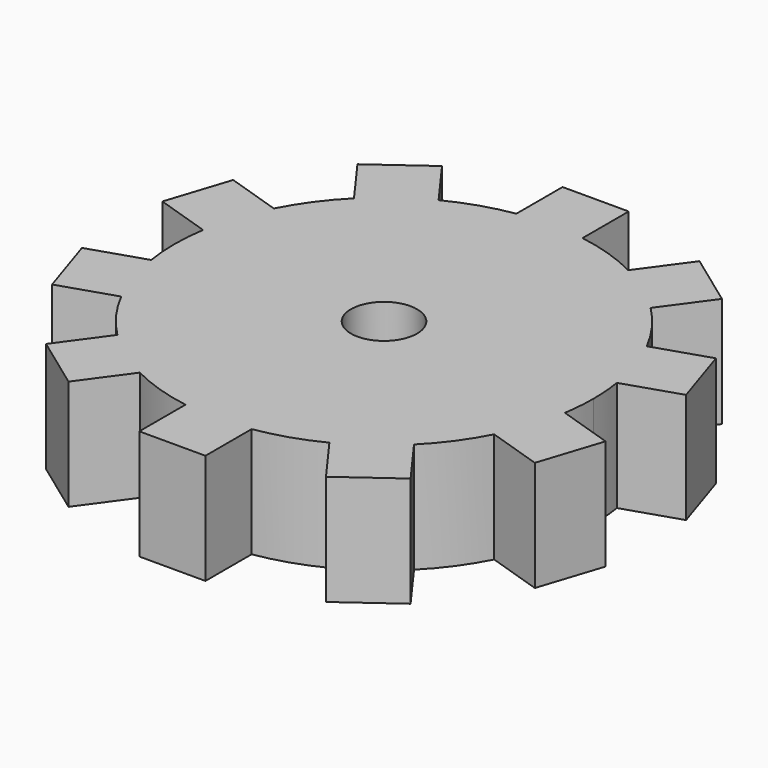
from build123d import *

# Parameters (mm, degrees)
F1_DEPTH = 12.7
F2_R     = 3.81
F3_DEPTH = 25.4


# Not quite as in the source:
# - a feature names something its author has since deleted; it is built from what else it names


with BuildPart() as f1:
    # F0 (on Top) → F1 (new body)
    with BuildSketch(Plane.XY):
        with BuildLine():
            ThreePointArc((23.8384751489, -3.7395190297), (24.0570083899, -1.8754325709), (24.13, 0))
            ThreePointArc((24.13, 0), (24.0570083899, 1.8754325709), (23.8384751489, 3.7395190297))
            Line((23.8384751489, 3.7395190297), (12.3294189943, 0))
            Line((12.3294189943, 0), (23.8384751489, -3.7395190297))
        make_face()
        with BuildLine():
            Line((12.3294189943, 0), (23.8384751489, 3.7395190297))
            ThreePointArc((23.8384751489, 3.7395190297), (22.9489937382, 7.4565800743), (21.4837656518, 10.9865696839))
            Line((21.4837656518, 10.9865696839), (9.9747094971, 7.2470506542))
            Line((9.9747094971, 7.2470506542), (6.1647094971, 2.0030355372))
            Line((6.1647094971, 2.0030355372), (12.3294189943, 0))
        make_face()
        with BuildLine():
            ThreePointArc((21.4837656518, 10.9865696839), (22.9489937382, 7.4565800743), (23.8384751489, 3.7395190297))
            Line((23.8384751489, 3.7395190297), (30.1655573652, 5.7953126615))
            Line((30.1655573652, 5.7953126615), (27.8108478681, 13.0423633156))
            Line((27.8108478681, 13.0423633156), (21.4837656518, 10.9865696839))
        make_face()
        with BuildLine():
            Line((30.1655573652, -5.7953126615), (23.8384751489, -3.7395190297))
            ThreePointArc((23.8384751489, -3.7395190297), (22.9489937382, -7.4565800743), (21.4837656518, -10.9865696839))
            Line((21.4837656518, -10.9865696839), (27.8108478681, -13.0423633156))
            Line((27.8108478681, -13.0423633156), (30.1655573652, -5.7953126615))
        make_face()
        with BuildLine():
            ThreePointArc((21.4837656518, -10.9865696839), (22.9489937382, -7.4565800743), (23.8384751489, -3.7395190297))
            Line((23.8384751489, -3.7395190297), (12.3294189943, 0))
            Line((12.3294189943, 0), (6.1647094971, -2.0030355372))
            Line((6.1647094971, -2.0030355372), (9.9747094971, -7.2470506542))
            Line((9.9747094971, -7.2470506542), (21.4837656518, -10.9865696839))
        make_face()
        with BuildLine():
            Line((9.9747094971, 7.2470506542), (21.4837656518, 10.9865696839))
            ThreePointArc((21.4837656518, 10.9865696839), (19.5215800743, 14.1832581378), (17.0876973792, 17.0372385755))
            Line((17.0876973792, 17.0372385755), (9.9747094971, 7.2470506542))
        make_face()
        with BuildLine():
            ThreePointArc((17.0876973792, -17.0372385755), (19.5215800743, -14.1832581378), (21.4837656518, -10.9865696839))
            Line((21.4837656518, -10.9865696839), (9.9747094971, -7.2470506542))
            Line((9.9747094971, -7.2470506542), (17.0876973792, -17.0372385755))
        make_face()
        with BuildLine():
            Line((9.9747094971, 7.2470506542), (17.0876973792, 17.0372385755))
            ThreePointArc((17.0876973792, 17.0372385755), (14.1832581378, 19.5215800743), (10.922987882, 21.516162198))
            Line((10.922987882, 21.516162198), (3.81, 11.7259742766))
            Line((3.81, 11.7259742766), (3.81, 5.244015117))
            Line((3.81, 5.244015117), (9.9747094971, 7.2470506542))
        make_face()
        with BuildLine():
            ThreePointArc((10.922987882, 21.516162198), (14.1832581378, 19.5215800743), (17.0876973792, 17.0372385755))
            Line((17.0876973792, 17.0372385755), (20.9980492384, 22.4193761773))
            Line((20.9980492384, 22.4193761773), (14.8333397413, 26.8982997998))
            Line((14.8333397413, 26.8982997998), (10.922987882, 21.516162198))
        make_face()
        with BuildLine():
            Line((20.9980492384, -22.4193761773), (17.0876973792, -17.0372385755))
            ThreePointArc((17.0876973792, -17.0372385755), (14.1832581378, -19.5215800743), (10.922987882, -21.516162198))
            Line((10.922987882, -21.516162198), (14.8333397413, -26.8982997998))
            Line((14.8333397413, -26.8982997998), (20.9980492384, -22.4193761773))
        make_face()
        with BuildLine():
            ThreePointArc((10.922987882, -21.516162198), (14.1832581378, -19.5215800743), (17.0876973792, -17.0372385755))
            Line((17.0876973792, -17.0372385755), (9.9747094971, -7.2470506542))
            Line((9.9747094971, -7.2470506542), (3.81, -5.244015117))
            Line((3.81, -5.244015117), (3.81, -11.7259742766))
            Line((3.81, -11.7259742766), (10.922987882, -21.516162198))
        make_face()
        with BuildLine():
            Line((3.81, 11.7259742766), (10.922987882, 21.516162198))
            ThreePointArc((10.922987882, 21.516162198), (7.4565800743, 22.9489937382), (3.81, 23.8273120599))
            Line((3.81, 23.8273120599), (3.81, 11.7259742766))
        make_face()
        with BuildLine():
            ThreePointArc((3.81, -23.8273120599), (7.4565800743, -22.9489937382), (10.922987882, -21.516162198))
            Line((10.922987882, -21.516162198), (3.81, -11.7259742766))
            Line((3.81, -11.7259742766), (3.81, -23.8273120599))
        make_face()
        with BuildLine():
            Line((3.81, 11.7259742766), (3.81, 23.8273120599))
            ThreePointArc((3.81, 23.8273120599), (0, 24.13), (-3.81, 23.8273120599))
            Line((-3.81, 23.8273120599), (-3.81, 11.7259742766))
            Line((-3.81, 11.7259742766), (0, 6.4819591596))
            Line((0, 6.4819591596), (3.81, 11.7259742766))
        make_face()
        with BuildLine():
            ThreePointArc((-3.81, 23.8273120599), (0, 24.13), (3.81, 23.8273120599))
            Line((3.81, 23.8273120599), (3.81, 30.48))
            Line((3.81, 30.48), (-3.81, 30.48))
            Line((-3.81, 30.48), (-3.81, 23.8273120599))
        make_face()
        with BuildLine():
            Line((3.81, -30.48), (3.81, -23.8273120599))
            ThreePointArc((3.81, -23.8273120599), (0, -24.13), (-3.81, -23.8273120599))
            Line((-3.81, -23.8273120599), (-3.81, -30.48))
            Line((-3.81, -30.48), (3.81, -30.48))
        make_face()
        with BuildLine():
            ThreePointArc((-3.81, -23.8273120599), (0, -24.13), (3.81, -23.8273120599))
            Line((3.81, -23.8273120599), (3.81, -11.7259742766))
            Line((3.81, -11.7259742766), (0, -6.4819591596))
            Line((0, -6.4819591596), (-3.81, -11.7259742766))
            Line((-3.81, -11.7259742766), (-3.81, -23.8273120599))
        make_face()
        with BuildLine():
            Line((-3.81, 11.7259742766), (-3.81, 23.8273120599))
            ThreePointArc((-3.81, 23.8273120599), (-7.4565800743, 22.9489937382), (-10.922987882, 21.516162198))
            Line((-10.922987882, 21.516162198), (-3.81, 11.7259742766))
        make_face()
        with BuildLine():
            ThreePointArc((-10.922987882, -21.516162198), (-7.4565800743, -22.9489937382), (-3.81, -23.8273120599))
            Line((-3.81, -23.8273120599), (-3.81, -11.7259742766))
            Line((-3.81, -11.7259742766), (-10.922987882, -21.516162198))
        make_face()
        with BuildLine():
            Line((-3.81, 11.7259742766), (-10.922987882, 21.516162198))
            ThreePointArc((-10.922987882, 21.516162198), (-14.1832581378, 19.5215800743), (-17.0876973792, 17.0372385755))
            Line((-17.0876973792, 17.0372385755), (-9.9747094971, 7.2470506542))
            Line((-9.9747094971, 7.2470506542), (-3.81, 5.244015117))
            Line((-3.81, 5.244015117), (-3.81, 11.7259742766))
        make_face()
        with BuildLine():
            ThreePointArc((-17.0876973792, 17.0372385755), (-14.1832581378, 19.5215800743), (-10.922987882, 21.516162198))
            Line((-10.922987882, 21.516162198), (-14.8333397413, 26.8982997998))
            Line((-14.8333397413, 26.8982997998), (-20.9980492384, 22.4193761773))
            Line((-20.9980492384, 22.4193761773), (-17.0876973792, 17.0372385755))
        make_face()
        with BuildLine():
            Line((-14.8333397413, -26.8982997998), (-10.922987882, -21.516162198))
            ThreePointArc((-10.922987882, -21.516162198), (-14.1832581378, -19.5215800743), (-17.0876973792, -17.0372385755))
            Line((-17.0876973792, -17.0372385755), (-20.9980492384, -22.4193761773))
            Line((-20.9980492384, -22.4193761773), (-14.8333397413, -26.8982997998))
        make_face()
        with BuildLine():
            ThreePointArc((-17.0876973792, -17.0372385755), (-14.1832581378, -19.5215800743), (-10.922987882, -21.516162198))
            Line((-10.922987882, -21.516162198), (-3.81, -11.7259742766))
            Line((-3.81, -11.7259742766), (-3.81, -5.244015117))
            Line((-3.81, -5.244015117), (-9.9747094971, -7.2470506542))
            Line((-9.9747094971, -7.2470506542), (-17.0876973792, -17.0372385755))
        make_face()
        with BuildLine():
            Line((-9.9747094971, 7.2470506542), (-17.0876973792, 17.0372385755))
            ThreePointArc((-17.0876973792, 17.0372385755), (-19.5215800743, 14.1832581378), (-21.4837656518, 10.9865696839))
            Line((-21.4837656518, 10.9865696839), (-9.9747094971, 7.2470506542))
        make_face()
        with BuildLine():
            ThreePointArc((-21.4837656518, -10.9865696839), (-19.5215800743, -14.1832581378), (-17.0876973792, -17.0372385755))
            Line((-17.0876973792, -17.0372385755), (-9.9747094971, -7.2470506542))
            Line((-9.9747094971, -7.2470506542), (-21.4837656518, -10.9865696839))
        make_face()
        with BuildLine():
            Line((-9.9747094971, 7.2470506542), (-21.4837656518, 10.9865696839))
            ThreePointArc((-21.4837656518, 10.9865696839), (-22.9489937382, 7.4565800743), (-23.8384751489, 3.7395190297))
            Line((-23.8384751489, 3.7395190297), (-12.3294189943, 0))
            Line((-12.3294189943, 0), (-6.1647094971, 2.0030355372))
            Line((-6.1647094971, 2.0030355372), (-9.9747094971, 7.2470506542))
        make_face()
        with BuildLine():
            ThreePointArc((-23.8384751489, 3.7395190297), (-22.9489937382, 7.4565800743), (-21.4837656518, 10.9865696839))
            Line((-21.4837656518, 10.9865696839), (-27.8108478681, 13.0423633156))
            Line((-27.8108478681, 13.0423633156), (-30.1655573652, 5.7953126615))
            Line((-30.1655573652, 5.7953126615), (-23.8384751489, 3.7395190297))
        make_face()
        with BuildLine():
            Line((-27.8108478681, -13.0423633156), (-21.4837656518, -10.9865696839))
            ThreePointArc((-21.4837656518, -10.9865696839), (-22.9489937382, -7.4565800743), (-23.8384751489, -3.7395190297))
            Line((-23.8384751489, -3.7395190297), (-30.1655573652, -5.7953126615))
            Line((-30.1655573652, -5.7953126615), (-27.8108478681, -13.0423633156))
        make_face()
        with BuildLine():
            ThreePointArc((-23.8384751489, -3.7395190297), (-22.9489937382, -7.4565800743), (-21.4837656518, -10.9865696839))
            Line((-21.4837656518, -10.9865696839), (-9.9747094971, -7.2470506542))
            Line((-9.9747094971, -7.2470506542), (-6.1647094971, -2.0030355372))
            Line((-6.1647094971, -2.0030355372), (-12.3294189943, 0))
            Line((-12.3294189943, 0), (-23.8384751489, -3.7395190297))
        make_face()
        with BuildLine():
            Line((-12.3294189943, 0), (-23.8384751489, 3.7395190297))
            ThreePointArc((-23.8384751489, 3.7395190297), (-24.13, 0), (-23.8384751489, -3.7395190297))
            Line((-23.8384751489, -3.7395190297), (-12.3294189943, 0))
        make_face()
        Polygon((0, -6.4819591596), (1.4552905029, -4.4789236225), (0, -4.0060710743), (-1.4552905029, -4.4789236225), align=None)
        Polygon((-3.81, -5.244015117), (-1.4552905029, -4.4789236225), (-2.3547094971, -3.2409795798), (-3.81, -2.7681270317), align=None)
        Polygon((-3.81, -2.7681270317), (-3.81, -1.2379440426), (-4.7094189943, 0), (-6.1647094971, -2.0030355372), align=None)
        Polygon((-3.81, 1.2379440426), (-3.81, 2.7681270317), (-6.1647094971, 2.0030355372), (-4.7094189943, 0), align=None)
        Polygon((3.81, -5.244015117), (3.81, -2.7681270317), (2.3547094971, -3.2409795798), (1.4552905029, -4.4789236225), align=None)
        Polygon((3.81, -2.7681270317), (6.1647094971, -2.0030355372), (4.7094189943, 0), (3.81, -1.2379440426), align=None)
        Polygon((6.1647094971, -2.0030355372), (12.3294189943, 0), (6.1647094971, 2.0030355372), (4.7094189943, 0), align=None)
        Polygon((9.9747094971, -7.2470506542), (6.1647094971, -2.0030355372), (3.81, -2.7681270317), (3.81, -5.244015117), align=None)
        Polygon((2.3547094971, -3.2409795798), (3.81, -2.7681270317), (3.81, -1.2379440426), (3.0823547486, -2.2394618112), align=None)
        Polygon((3.81, -11.7259742766), (3.81, -5.244015117), (1.4552905029, -4.4789236225), (0, -6.4819591596), align=None)
        Polygon((1.4552905029, -4.4789236225), (2.3547094971, -3.2409795798), (1.1773547486, -3.6235253271), (0, -4.0060710743), align=None)
        Polygon((-3.81, -11.7259742766), (0, -6.4819591596), (-1.4552905029, -4.4789236225), (-3.81, -5.244015117), align=None)
        Polygon((-1.4552905029, -4.4789236225), (0, -4.0060710743), (-1.1773547486, -3.6235253271), (-2.3547094971, -3.2409795798), align=None)
        Polygon((-9.9747094971, -7.2470506542), (-3.81, -5.244015117), (-3.81, -2.7681270317), (-6.1647094971, -2.0030355372), align=None)
        Polygon((-3.81, -2.7681270317), (-2.3547094971, -3.2409795798), (-3.0823547486, -2.2394618112), (-3.81, -1.2379440426), align=None)
        Polygon((-4.7094189943, 0), (-6.1647094971, 2.0030355372), (-12.3294189943, 0), (-6.1647094971, -2.0030355372), align=None)
        Polygon((-3.81, -1.2379440426), (-3.81, 0), (-3.81, 1.2379440426), (-4.7094189943, 0), align=None)
        Polygon((-3.81, 2.7681270317), (-3.81, 5.244015117), (-9.9747094971, 7.2470506542), (-6.1647094971, 2.0030355372), align=None)
        Polygon((-3.0823547486, 2.2394618112), (-2.3547094971, 3.2409795798), (-3.81, 2.7681270317), (-3.81, 1.2379440426), align=None)
        Polygon((-1.4552905029, 4.4789236225), (0, 6.4819591596), (-3.81, 11.7259742766), (-3.81, 5.244015117), align=None)
        Polygon((-2.3547094971, 3.2409795798), (-1.4552905029, 4.4789236225), (-3.81, 5.244015117), (-3.81, 2.7681270317), align=None)
        Polygon((6.1647094971, 2.0030355372), (9.9747094971, 7.2470506542), (3.81, 5.244015117), (3.81, 2.7681270317), align=None)
        Polygon((1.4552905029, 4.4789236225), (3.81, 5.244015117), (3.81, 11.7259742766), (0, 6.4819591596), align=None)
        Polygon((-1.1773547486, 3.6235253271), (0, 4.0060710743), (-1.4552905029, 4.4789236225), (-2.3547094971, 3.2409795798), align=None)
        Polygon((0, 4.0060710743), (1.4552905029, 4.4789236225), (0, 6.4819591596), (-1.4552905029, 4.4789236225), align=None)
        Polygon((2.3547094971, 3.2409795798), (1.4552905029, 4.4789236225), (0, 4.0060710743), (1.1773547486, 3.6235253271), align=None)
        Polygon((3.81, 1.2379440426), (3.81, 2.7681270317), (2.3547094971, 3.2409795798), (3.0823547486, 2.2394618112), align=None)
        Polygon((4.7094189943, 0), (6.1647094971, 2.0030355372), (3.81, 2.7681270317), (3.81, 1.2379440426), align=None)
        Polygon((3.81, -1.2379440426), (4.7094189943, 0), (3.81, 1.2379440426), (3.81, 0), align=None)
        Polygon((3.81, 2.7681270317), (3.81, 5.244015117), (1.4552905029, 4.4789236225), (2.3547094971, 3.2409795798), align=None)
        Polygon((3.81, 0), (3.81, 1.2379440426), (3.0823547486, 2.2394618112), (2.3547094971, 3.2409795798), (1.1773547486, 3.6235253271), (0, 4.0060710743), (-1.1773547486, 3.6235253271), (-2.3547094971, 3.2409795798), (-3.0823547486, 2.2394618112), (-3.81, 1.2379440426), (-3.81, 0), (0, 0), align=None)
        Polygon((3.0823547486, -2.2394618112), (3.81, -1.2379440426), (3.81, 0), (0, 0), (-3.81, 0), (-3.81, -1.2379440426), (-3.0823547486, -2.2394618112), (-2.3547094971, -3.2409795798), (-1.1773547486, -3.6235253271), (0, -4.0060710743), (1.1773547486, -3.6235253271), (2.3547094971, -3.2409795798), align=None)
    extrude(amount=F1_DEPTH)

    # F2 (on face) → F3 (cut)
    with BuildSketch(Plane.XY.offset(12.7)):
        Circle(F2_R)
    extrude(amount=-F3_DEPTH, mode=Mode.SUBTRACT)


solid = f1.part
